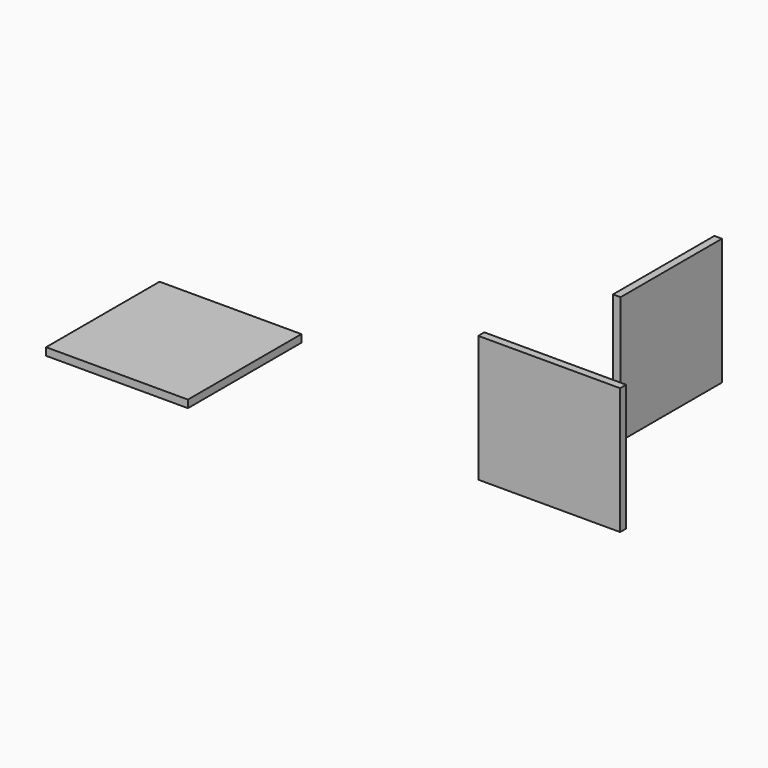
from build123d import *

# Parameters (mm, degrees)
F1_W     = 88.9
F1_H     = 79.375
F2_DEPTH = 2.38125
F3_W     = 79.375
F3_H     = 79.375
F4_DEPTH = 2.38125
F5_W     = 88.9
F5_H     = 88.9
F6_DEPTH = 2.38125


# Not quite as in the source:
# - a variable given as a bare number and used for a length is read in inches; the dataset says mm whatever the document's units were


with BuildPart() as f2:
    # F1 (on Front) → F2 (new body, symmetric)
    with BuildSketch(Plane.XZ):
        Rectangle(F1_W, F1_H)
    extrude(amount=F2_DEPTH, both=True)


with BuildPart() as f4:
    # F3 (on Right) → F4 (new body, symmetric)
    with BuildSketch(Plane.YZ):
        with Locations((90.2850845814, 15.0111026208)):
            Rectangle(F3_W, F3_H)
    extrude(amount=F4_DEPTH, both=True)


with BuildPart() as f6:
    # F5 (on Top) → F6 (new body, symmetric)
    with BuildSketch(Plane.XY):
        with Locations((-202.4036215127, -43.4954859122)):
            Rectangle(F5_W, F5_H)
    extrude(amount=F6_DEPTH, both=True)


solid = Compound([f2.part, f4.part, f6.part])
